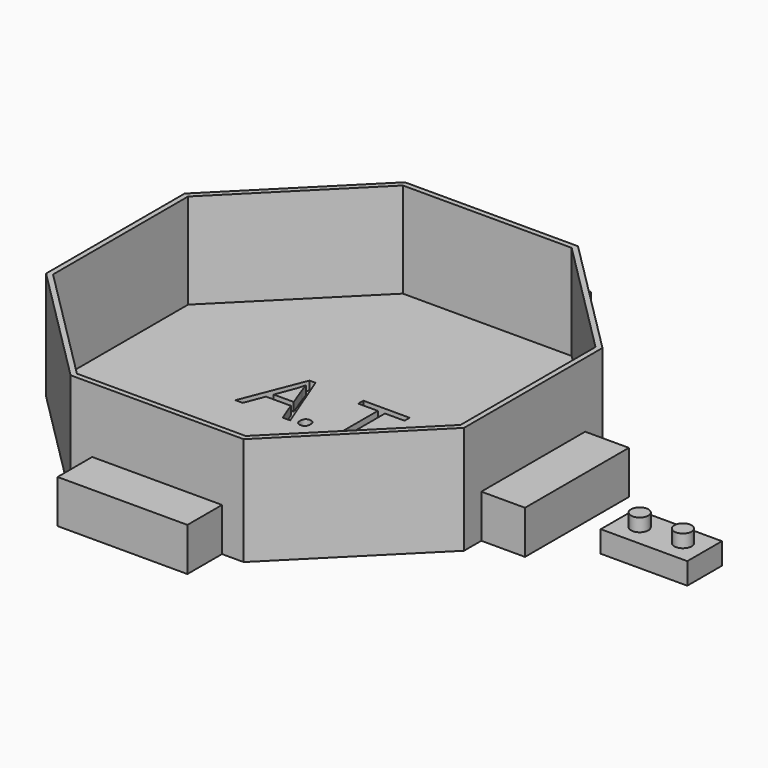
from build123d import *

# Parameters (mm, degrees)
F0_W          = 20
F0_H          = 10
F1_DEPTH      = 5
F2_R          = 2
F3_DEPTH      = 3
F5_DEPTH      = 25
F6_DEPTH      = 5
F7_R          = 2
F8_DEPTH      = 3
F11_W         = 30
F11_H         = 10
F12_DEPTH     = 10
F10_W         = 30
F10_H         = 10
F13_DEPTH     = 10.1
F9_W          = 30
F9_H          = 10
F14_DEPTH     = 10
F16_DEPTH     = 22
F17_TEXT_SIZE = 19.9860752645
F18_DEPTH     = 2


# Not quite as in the source:
# - Text() gives the source's letters only with a copy of the font that has no kerning and outlines rounded to 1/6400 em; it was checked with that copy


with BuildPart() as f1:
    # F0 (on Top) → F1 (new body)
    with BuildSketch(Plane.XY):
        with Locations((6.0114492662, -0.4977477107)):
            Rectangle(F0_W, F0_H)
    extrude(amount=F1_DEPTH)

    # F2 (on face) → F3 (join)
    with BuildSketch(Plane.XY.offset(5)):
        with Locations((1.0114492662, -0.4977477107)):
            Circle(F2_R)
        with Locations((11.0114492662, -0.4977477107)):
            Circle(F2_R)
    extrude(amount=F3_DEPTH)


with BuildPart() as f5:
    # F4 (on Top) → F5 (new body)
    with BuildSketch(Plane.XY):
        Polygon((-52.2728219812, -48.2842712475), (-23.9885507338, -20), (-23.9885507338, 20), (-52.2728219812, 48.2842712475), (-92.2728219812, 48.2842712475), (-120.5570932287, 20), (-120.5570932287, 5), (-120.5570932287, -1.0517463742), (-120.5570932287, -5), (-120.5570932287, -11.0517463742), (-120.5570932287, -20), (-92.2728219812, -48.2842712475), align=None)
    extrude(amount=F5_DEPTH)

    # F4 (on Top) → F6 (join)
    with BuildSketch(Plane.XY):
        Polygon((-130.5570932287, -5), (-120.5570932287, -5), (-120.5570932287, -1.0517463742), (-120.5570932287, 5), (-130.5570932287, 5), align=None)
    extrude(amount=F6_DEPTH)

    # F7 (on face) → F8 (cut)
    with BuildSketch(Plane.XY.offset(5)):
        with Locations((-125.5570932287, 0)):
            Circle(F7_R)
    extrude(amount=-F8_DEPTH, mode=Mode.SUBTRACT)

    # F11 (on face) → F12 (join)
    with BuildSketch(Plane(origin=(0, 48.2842712475, 0), x_dir=(-1, 0, 0), z_dir=(0, 1, 0))):
        with Locations((72.2728219812, 5)):
            Rectangle(F11_W, F11_H)
    extrude(amount=F12_DEPTH)

    # F10 (on face) → F13 (join)
    with BuildSketch(Plane.YZ.offset(-23.9885507338)):
        with Locations((0, 5)):
            Rectangle(F10_W, F10_H)
    extrude(amount=F13_DEPTH)

    # F9 (on face) → F14 (join)
    with BuildSketch(Plane.XZ.offset(48.2842712475)):
        with Locations((-72.2728219812, 5)):
            Rectangle(F9_W, F9_H)
    extrude(amount=F14_DEPTH)

    # F15 (on face) → F16 (cut)
    with BuildSketch(Plane.XY.offset(25)):
        Polygon((-91.7728219812, -47.0771644663), (-52.7728219812, -47.0771644663), (-25.195657515, -19.5), (-25.195657515, 19.5), (-52.7728219812, 47.0771644663), (-91.7728219812, 47.0771644663), (-119.3499864475, 19.5), (-119.3499864475, -19.5), align=None)
    extrude(amount=-F16_DEPTH, mode=Mode.SUBTRACT)

    # F17 (on face) → F18 (cut)
    with BuildSketch(Plane.XY.offset(3)):
        with Locations((-89.3499864475, -4.3128097242)):
            Text('A.T.', F17_TEXT_SIZE, font='Open Sans', text_align=(TextAlign.LEFT, TextAlign.BOTTOM))
    extrude(amount=-F18_DEPTH, mode=Mode.SUBTRACT)


solid = Compound([f1.part, f5.part])
